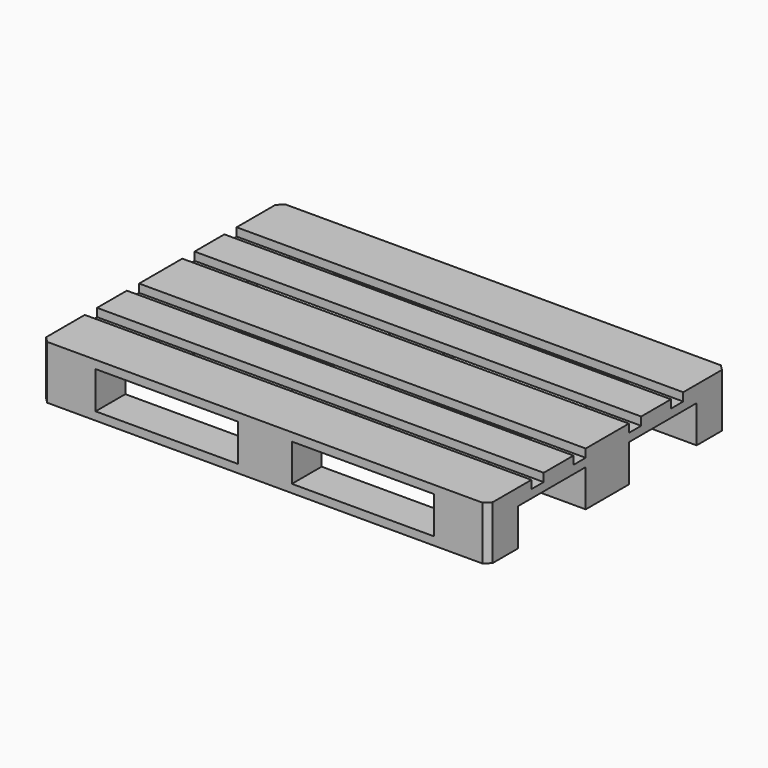
from build123d import *

# Parameters (mm, degrees)
F0_W     = 1200
F0_H     = 145
F1_DEPTH = 22
F0_H_2   = 100
F2_W     = 145
F2_H     = 655
F2_H_2   = 145
F3_DEPTH = 22
F4_W     = 145
F4_H     = 100
F4_H_2   = 145
F5_W     = 145
F5_H     = 145
F5_H_2   = 100
F6_DEPTH = 78
F7_W     = 145
F7_H     = 100
F7_W_2   = 1055
F7_W_3   = 1200
F7_H_2   = 145
F8_DEPTH = 22
F9_SIZE  = 15


# Not quite as in the source:
# - a feature names something its author has since deleted; it is built from what else it names


with BuildPart() as f1:
    # F0 (on Top) → F1 (new body)
    with BuildSketch(Plane.XY):
        with Locations((0, 327.5)):
            Rectangle(F0_W, F0_H)
    extrude(amount=-F1_DEPTH)



with BuildPart() as f1b:
    # F0 (on Top) → F1, piece 2 (new body)
    with BuildSketch(Plane.XY):
        with Locations((0, 163.75)):
            Rectangle(F0_W, F0_H_2)
    extrude(amount=-F1_DEPTH)


with BuildPart() as f1c:
    # F0 (on Top) → F1, piece 3 (new body)
    with BuildSketch(Plane.XY):
        Rectangle(F0_W, F0_H)
    extrude(amount=-F1_DEPTH)


with BuildPart() as f1d:
    # F0 (on Top) → F1, piece 4 (new body)
    with BuildSketch(Plane.XY):
        with Locations((0, -163.75)):
            Rectangle(F0_W, F0_H_2)
    extrude(amount=-F1_DEPTH)


with BuildPart() as f1e:
    # F0 (on Top) → F1, piece 5 (new body)
    with BuildSketch(Plane.XY):
        with Locations((0, -327.5)):
            Rectangle(F0_W, F0_H)
    extrude(amount=-F1_DEPTH)


with BuildPart() as f1_1:
    add(f1.part)

    add(f1b.part)  # F3 merges F1b

    add(f1c.part)  # F3 merges F1c

    add(f1d.part)  # F3 merges F1d

    add(f1e.part)  # F3 merges F1e
    # F2 (on face) → F3 (join)
    with BuildSketch(Plane(origin=(0, 0, -22), x_dir=(1, 0, 0), z_dir=(0, 0, -1))):
        with Locations((-527.5, -72.5)):
            Rectangle(F2_W, F2_H)
        with Locations((-527.5, 327.5)):
            Rectangle(F2_W, F2_H_2)
        with Locations((0, 327.5)):
            Rectangle(F2_W, F2_H_2)
        with Locations((0, -72.5)):
            Rectangle(F2_W, F2_H)
        with Locations((527.5, 327.5)):
            Rectangle(F2_W, F2_H_2)
        with Locations((527.5, -72.5)):
            Rectangle(F2_W, F2_H)
    extrude(amount=F3_DEPTH)

    # F4 (on face) + F5 (on face) → F6 (join)
    with BuildSketch(Plane(origin=(0, 0, -44), x_dir=(1, 0, 0), z_dir=(0, 0, -1))):
        with Locations((-527.5, -350)):
            Rectangle(F4_W, F4_H)
        with Locations((-527.5, 350)):
            Rectangle(F4_W, F4_H)
        with Locations((527.5, -350)):
            Rectangle(F4_W, F4_H)
        with Locations((527.5, 0)):
            Rectangle(F4_W, F4_H_2)
        with Locations((527.5, 350)):
            Rectangle(F4_W, F4_H)
        with Locations((-527.5, 0)):
            Rectangle(F4_W, F4_H_2)
    with BuildSketch(Plane(origin=(0, 0, -44), x_dir=(1, 0, 0), z_dir=(0, 0, -1))):
        Rectangle(F5_W, F5_H)
        with Locations((0, 350)):
            Rectangle(F5_W, F5_H_2)
        with Locations((0, -350)):
            Rectangle(F5_W, F5_H_2)
    extrude(amount=F6_DEPTH)

    # F7 (on face) → F8 (join)
    with BuildSketch(Plane(origin=(0, 0, -122), x_dir=(1, 0, 0), z_dir=(0, 0, -1))):
        with Locations((-527.5, -350)):
            Rectangle(F7_W, F7_H)
        with Locations((72.5, -350)):
            Rectangle(F7_W_2, F7_H)
        Rectangle(F7_W_3, F7_H_2)
        with Locations((0, 350)):
            Rectangle(F7_W_3, F7_H)
    extrude(amount=F8_DEPTH)

    # F9
    f9_edges = [f1_1.edges().sort_by_distance(p)[0] for p in [
        (-600, -400, -72),
        (600, -400, -72),
        (600, 400, -72),
        (-600, 400, -72),
    ]]
    chamfer(f9_edges, length=F9_SIZE)


solid = f1_1.part
